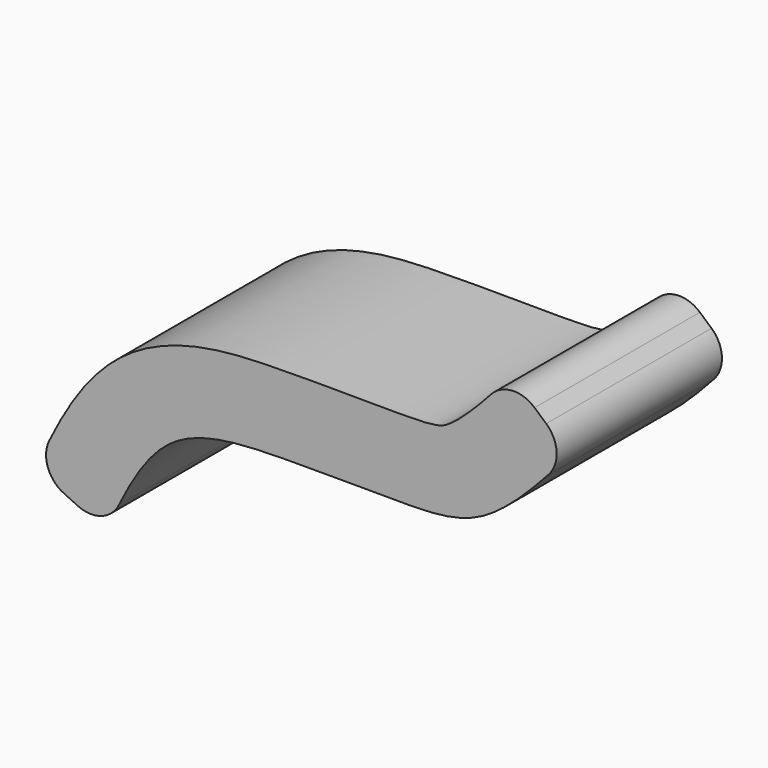
from build123d import *

# Parameters (mm, degrees)
F1_DEPTH = 50.8
F2_R     = 7.62


# Not quite as in the source:
# - the dataset's text gives a spline's control points without its knots; the knots are read off the source's solid


with BuildPart() as f1:
    # F0 (on Front) → F1 (new body)
    with BuildSketch(Plane.XZ):
        with BuildLine():
            Line((-59.3070761655, -21.8227360142), (-42.0378260314, -29.8648439348))
            add(Edge.make_bspline(
                [(-42.0378260314, -29.8648439348), (-37.5408292143, -20.2082012168), (-28.7610191004, -1.3548435544), (0.1852591164, 0.4500649959), (31.4439243402, -0.3003332078), (51.7274502596, 0.7006149211), (64.7157226613, 15.3713666937), (71.9278976321, 23.5177949071)],
                knots=[0, 0, 0, 0, 0.2081160567, 0.4063199361, 0.6231846725, 0.7907606193, 1, 1, 1, 1], degree=3))
            Line((71.9278976321, 23.5177949071), (57.66448368, 36.1454440324))
            add(Edge.make_bspline(
                [(-59.3070761655, -21.8227360142), (-58.631822402, -20.372727352), (-57.2326609344, -17.3669870215), (-54.9195750463, -12.6269553993), (-52.290883787, -7.7265549055), (-49.7175719467, -3.561686059), (-47.3279051008, -0.2220423536), (-45.338427998, 2.2702424421), (-43.1183370493, 4.7275950198), (-41.0477397791, 6.7190800232), (-39.2442762759, 8.2556682686), (-38.0539774048, 9.1862612918), (-37.0623497299, 9.9095055954), (-36.0465553439, 10.6154075646), (-34.7650769471, 11.4423890704), (-33.2084485385, 12.3527532604), (-31.1196933377, 13.458167234), (-27.4494612164, 15.1196460437), (-22.2727789213, 16.7917213418), (-16.3376615725, 17.9817161001), (-11.6469124365, 18.5203096146), (-8.0400800968, 18.7814841119), (-5.4053373413, 18.9124255501), (-3.2675723307, 18.982544513), (-1.5906986648, 19.0230733609), (-0.3526104933, 19.0474071732), (0.87734965, 19.0675835008), (2.5219132672, 19.0896147925), (4.5769506756, 19.1085778208), (7.0383090768, 19.1198065178), (10.3046004987, 19.1221708173), (14.3424252523, 19.1066043772), (19.0599234, 19.0741289863), (22.8345528238, 19.0483452659), (25.7277137641, 19.0358659389), (27.8251785593, 19.0323438017), (29.5058814233, 19.035692451), (30.8030558592, 19.0429376699), (31.7561028254, 19.0508346878), (32.6626871735, 19.0613596046), (33.8021161008, 19.0804572118), (35.0978461461, 19.1162037558), (36.4431452359, 19.1827126493), (37.5801812791, 19.2732225909), (38.515911426, 19.3839735558), (39.5173517276, 19.5506644088), (40.1985488805, 19.7285768595), (40.6670707589, 19.8958738921), (40.9265642367, 20.0036637108), (41.1234439392, 20.0935670417), (41.2950071187, 20.1792714123), (41.439100667, 20.2560871994), (41.603013776, 20.3470701295), (41.8399423013, 20.4860480773), (42.2834626322, 20.7648864981), (42.9477447613, 21.2208645946), (43.8912236782, 21.9391381184), (44.9557550555, 22.8214415778), (46.5092157464, 24.2027241023), (48.6592995414, 26.2830875471), (51.4782616603, 29.2395128834), (54.4816322492, 32.550604721), (56.5873419532, 34.9287711439), (57.66448368, 36.1454440324)],
                knots=[0, 0, 0, 0, 0.03125, 0.0625, 0.09375, 0.125, 0.140625, 0.15625, 0.171875, 0.1875, 0.1953125, 0.203125, 0.20703125, 0.2109375, 0.21875, 0.2265625, 0.234375, 0.25, 0.28125, 0.3125, 0.34375, 0.359375, 0.375, 0.390625, 0.3984375, 0.40625, 0.4140625, 0.421875, 0.4375, 0.453125, 0.46875, 0.5, 0.53125, 0.5625, 0.578125, 0.59375, 0.609375, 0.6171875, 0.625, 0.6328125, 0.640625, 0.65625, 0.671875, 0.6875, 0.703125, 0.71875, 0.75, 0.765625, 0.7734375, 0.78125, 0.7890625, 0.79296875, 0.796875, 0.8046875, 0.8125, 0.828125, 0.84375, 0.859375, 0.875, 0.90625, 0.9375, 0.96875, 1, 1, 1, 1], degree=3))
        make_face()
    extrude(amount=F1_DEPTH)

    # F2
    f2_edges = [f1.edges().sort_by_distance(p)[0] for p in [
        (57.664484, -25.4, 36.145444),
        (71.927898, -25.4, 23.517795),
        (-59.307076, -25.4, -21.822736),
        (-42.037826, -25.4, -29.864844),
    ]]
    fillet(f2_edges, radius=F2_R)


solid = f1.part
